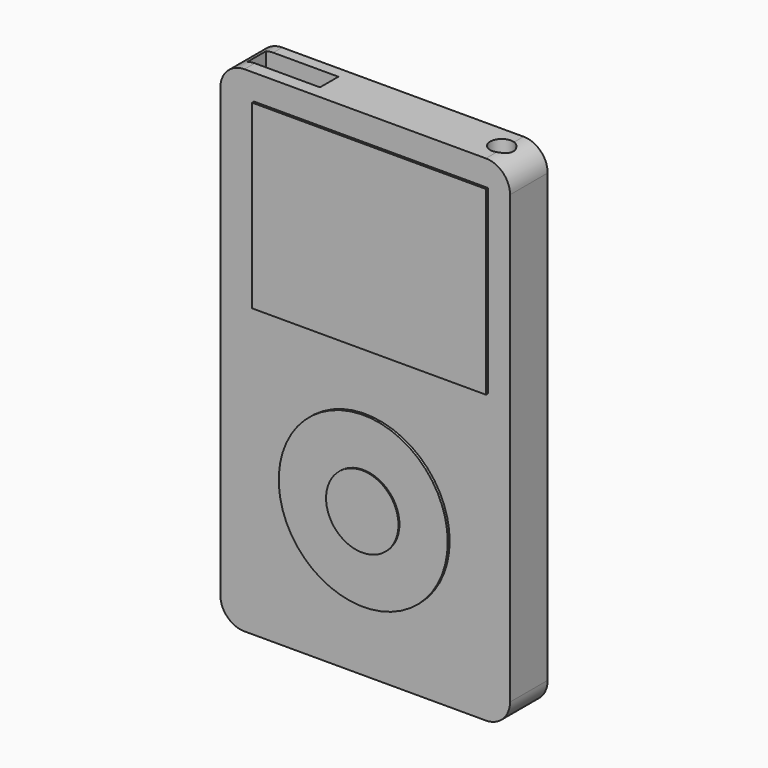
from build123d import *

# Parameters (mm, degrees)
F0_W        = 60.96
F0_H        = 104.14
F1_DEPTH    = 10.414
F2_W        = 60.96
F2_H        = 104.14
F2_R        = 17.78
F2_W_2      = 49.2147877812
F2_H_2      = 38.1
F3_DEPTH    = 0.508
F4_R        = 7.62
F5_DEPTH    = 0.254
F6_W        = 15.2469340246
F6_H        = 4.8402966931
F6_R        = 2.4201483466
F7_DEPTH    = 25.4
F8_T1_DEPTH = 35.306
F9_W        = 22.3395526409
F9_H        = 4.0701881517
F10_DEPTH   = 25.4


# Not quite as in the source:
# - a fillet or chamfer that OpenCascade refuses, or shapes differently, is made with other operations: its cross-section is extruded or revolved along the edge and cut away or added


with BuildPart() as f1:
    # F0 (on Front) → F1 (new body)
    with BuildSketch(Plane.XZ):
        with Locations((9.1376345801, 0.7195156068)):
            Rectangle(F0_W, F0_H)
    extrude(amount=F1_DEPTH)

    # F2 (on face) → F3 (cut)
    with BuildSketch(Plane.XZ.offset(10.414)):
        with Locations((9.1376345801, 0.7195156068)):
            Rectangle(F2_W, F2_H)
        with Locations((9.1376345801, -20.5781124532)):
            Circle(F2_R, mode=Mode.SUBTRACT)
        with Locations((10.3610083461, 28.4036870554)):
            Rectangle(F2_W_2, F2_H_2, mode=Mode.SUBTRACT)
    extrude(amount=-F3_DEPTH, mode=Mode.SUBTRACT)

    # F4 (on face) → F5 (join)
    with BuildSketch(Plane.XZ.offset(10.414)):
        with Locations((9.1376345801, -20.5781124532)):
            Circle(F4_R)
    extrude(amount=F5_DEPTH)

    # F6 (on face) → F7 (cut)
    with BuildSketch(Plane.XY.offset(52.7895156068)):
        with Locations((-10.1616705069, -4.773916211)):
            Rectangle(F6_W, F6_H)
        with Locations((33.7640233338, -4.773916211)):
            Circle(F6_R)
    extrude(amount=-F7_DEPTH, mode=Mode.SUBTRACT)

    # F8: fillet of radius 5.08 on 4 edges, made by hand

    # F8_s2 → F8_t1 (cut)
    with BuildSketch(Plane.XZ.offset(-12.7)):
        with BuildLine():
            ThreePointArc((39.6176345801, -46.2704843932), (38.1297370286, -49.8625868417), (34.5376345801, -51.3504843932))
            Line((34.5376345801, -51.3504843932), (39.6176345801, -51.3504843932))
            Line((39.6176345801, -51.3504843932), (39.6176345801, -46.2704843932))
        make_face()
        with BuildLine():
            ThreePointArc((-21.3423654199, -46.2704843932), (-19.8544678683, -49.8625868417), (-16.2623654199, -51.3504843932))
            Line((-16.2623654199, -51.3504843932), (-21.3423654199, -51.3504843932))
            Line((-21.3423654199, -51.3504843932), (-21.3423654199, -46.2704843932))
        make_face()
        with BuildLine():
            ThreePointArc((-16.2623654199, 52.7895156068), (-19.8544678683, 51.3016180552), (-21.3423654199, 47.7095156068))
            Line((-21.3423654199, 47.7095156068), (-21.3423654199, 52.7895156068))
            Line((-21.3423654199, 52.7895156068), (-16.2623654199, 52.7895156068))
        make_face()
        with BuildLine():
            ThreePointArc((34.5376345801, 52.7895156068), (38.1297370286, 51.3016180552), (39.6176345801, 47.7095156068))
            Line((39.6176345801, 47.7095156068), (39.6176345801, 52.7895156068))
            Line((39.6176345801, 52.7895156068), (34.5376345801, 52.7895156068))
        make_face()
    extrude(amount=F8_T1_DEPTH, mode=Mode.SUBTRACT)

    # F9 (on face) → F10 (cut)
    with BuildSketch(Plane(origin=(0, 0, -51.3504843932), x_dir=(1, 0, 0), z_dir=(0, 0, -1))):
        with Locations((11.1697763205, 4.9349990441)):
            Rectangle(F9_W, F9_H)
    extrude(amount=-F10_DEPTH, mode=Mode.SUBTRACT)


solid = f1.part
